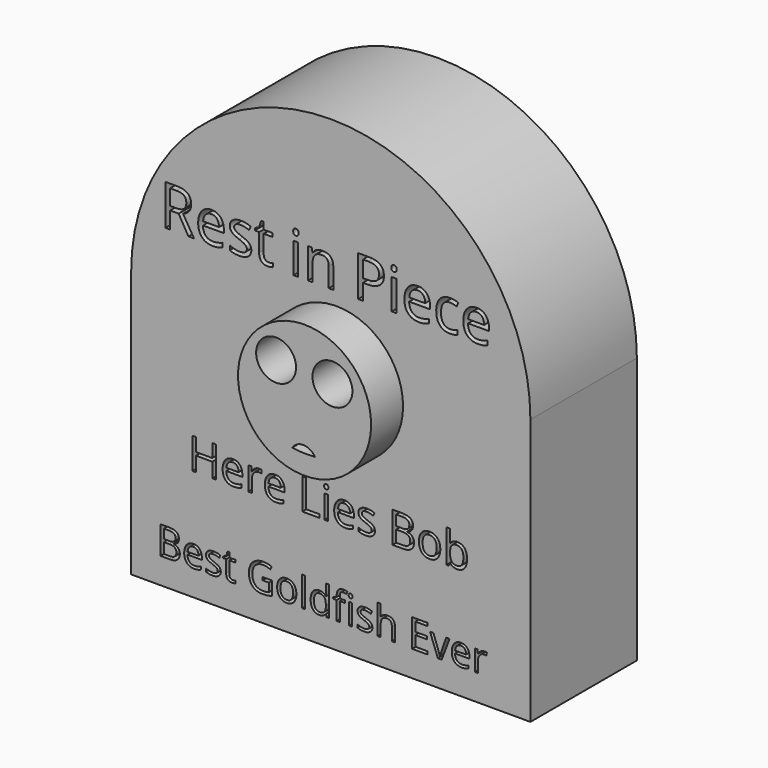
from build123d import *

# Parameters (mm, degrees)
F1_DEPTH       = 25.4
F2_TEXT_SIZE   = 10.8335776931
F2_TEXT_SIZE_2 = 8.309870221
F2_TEXT_SIZE_3 = 7.4563334801
F3_DEPTH       = 12.7
F4_R           = 12.7
F4_R_2         = 3.81
F5_DEPTH       = 7.62


# Not quite as in the source:
# - Text() gives the source's letters only with a copy of the font that has no kerning and outlines rounded to 1/6400 em; it was checked with that copy


with BuildPart() as f1:
    # F0 (on Front) → F1 (new body)
    with BuildSketch(Plane.XZ):
        with BuildLine():
            Line((-44.5170775056, 30.8612820968), (-44.5170775056, -19.9387179032))
            Line((-44.5170775056, -19.9387179032), (31.6829224944, -19.9387179032))
            Line((31.6829224944, -19.9387179032), (31.6829224944, 30.8612820968))
            ThreePointArc((31.6829224944, 30.8612820968), (-6.4170775056, 68.9612820968), (-44.5170775056, 30.8612820968))
        make_face()
    extrude(amount=F1_DEPTH)

    # F2 (on face) → F3 (cut)
    with BuildSketch(Plane.XZ.offset(25.4)):
        with Locations((-39.0268916986, 40.4149880241)):
            Text('Rest in Piece', F2_TEXT_SIZE, font='Open Sans', text_align=(TextAlign.LEFT, TextAlign.BOTTOM))
        with Locations((-33.6555754766, 1.2485745829)):
            Text('Here Lies Bob', F2_TEXT_SIZE_2, font='Open Sans', text_align=(TextAlign.LEFT, TextAlign.BOTTOM))
        with Locations((-39.6386766806, -14.9983619527)):
            Text('Best Goldfish Ever', F2_TEXT_SIZE_3, font='Open Sans', text_align=(TextAlign.LEFT, TextAlign.BOTTOM))
    extrude(amount=-F3_DEPTH, mode=Mode.SUBTRACT)

    # F4 (on face) → F5 (join)
    with BuildSketch(Plane.XZ.offset(25.4)):
        with Locations((-5.3204763681, 25.1868385822)):
            Circle(F4_R)
        with BuildLine():
            ThreePointArc((-3.3632934671, 16.3078687654), (-5.5261830893, 16.2429805241), (-7.6803940578, 16.4471302357))
            ThreePointArc((-7.6803940578, 16.4471302357), (-5.4830555501, 17.5799326925), (-3.3632934671, 16.3078687654))
        make_face(mode=Mode.SUBTRACT)
        with Locations((-10.7558348021, 30.1496200264)):
            Circle(F4_R_2, mode=Mode.SUBTRACT)
        with Locations((0, 29.6362284571)):
            Circle(F4_R_2, mode=Mode.SUBTRACT)
    extrude(amount=F5_DEPTH)


solid = f1.part
